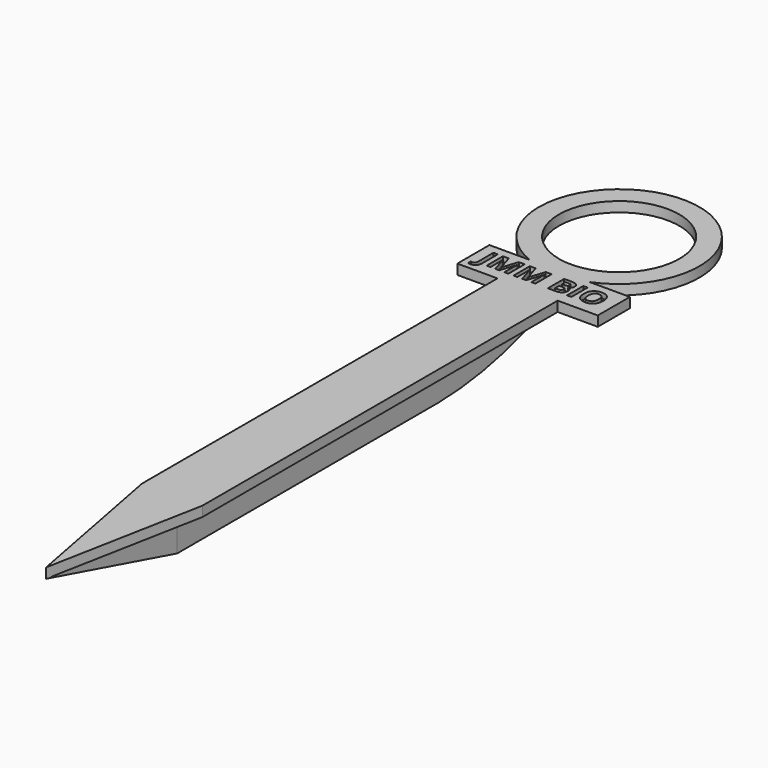
from build123d import *

# Parameters (mm, degrees)
F0_R         = 19.05
F1_DEPTH     = 3.175
F2_W         = 3.175
F2_H         = 153.3009581755
F3_DEPTH     = 12.7
F5_DEPTH     = 128.016
F6_W         = 12.7
F6_H         = 12.7
F7_DEPTH     = 3.175
F8_ANGLE     = 180
F9_TEXT_SIZE = 9.0372655213
F10_DEPTH    = 1.5875


# Not quite as in the source:
# - Text() gives the source's letters only with a copy of the font that has no kerning and outlines rounded to 1/6400 em; it was checked with that copy


with BuildPart() as f1:
    # F0 (on Top) → F1 (new body)
    with BuildSketch(Plane.XY):
        with BuildLine():
            ThreePointArc((-32.8058722675, 92.5149641021), (-42.3308722675, 90.6613942987), (-51.8558722675, 92.5149641021))
            Line((-51.8558722675, 92.5149641021), (-51.8558722675, -60.7859940734))
            Line((-51.8558722675, -60.7859940734), (-42.3308722675, -110.6850358979))
            Line((-42.3308722675, -110.6850358979), (-32.8058722675, -60.7859940734))
            Line((-32.8058722675, -60.7859940734), (-32.8058722675, 92.5149641021))
        make_face()
        with BuildLine():
            Line((-32.8058722675, 92.5149641021), (-51.8558722675, 92.5149641021))
            ThreePointArc((-51.8558722675, 92.5149641021), (-42.3308722675, 90.6613942987), (-32.8058722675, 92.5149641021))
        make_face()
        with BuildLine():
            ThreePointArc((-16.9308722675, 116.0613942987), (-56.5299039246, 137.1219617174), (-51.8558722675, 92.5149641021))
            Line((-51.8558722675, 92.5149641021), (-32.8058722675, 92.5149641021))
            ThreePointArc((-32.8058722675, 92.5149641021), (-21.2703048487, 101.8623626415), (-16.9308722675, 116.0613942987))
        make_face()
        with Locations((-42.3308722675, 116.0613942987)):
            Circle(F0_R, mode=Mode.SUBTRACT)
    extrude(amount=F1_DEPTH)

    # F2 (on face) → F3 (join)
    with BuildSketch(Plane.XY.offset(3.175)):
        with Locations((-42.3308722675, 15.8644850144)):
            Rectangle(F2_W, F2_H)
        Polygon((-40.7433722675, -60.7859940734), (-43.9183722675, -60.7859940734), (-42.3308722675, -110.6850358979), align=None)
    extrude(amount=F3_DEPTH)

    # F4 (on Right) → F5 (cut)
    with BuildSketch(Plane.YZ):
        Polygon((-110.6850358979, 3.175), (-60.7859940734, 15.875), (-110.6850358979, 15.875), align=None)
        with BuildLine():
            ThreePointArc((42.7295640111, 15.875), (68.363979336, 12.4326056643), (92.5149641021, 3.175))
            Line((92.5149641021, 3.175), (92.5149641021, 15.875))
            Line((92.5149641021, 15.875), (42.7295640111, 15.875))
        make_face()
    extrude(amount=-F5_DEPTH, mode=Mode.SUBTRACT)

    # F6 (on face) → F7 (join)
    with BuildSketch(Plane(origin=(0, 0, 0), x_dir=(1, 0, 0), z_dir=(0, 0, -1))):
        with Locations((-26.4558722675, -86.1649641021)):
            Rectangle(F6_W, F6_H)
        with Locations((-58.2058722675, -86.1649641021)):
            Rectangle(F6_W, F6_H)
    extrude(amount=-F7_DEPTH)


with BuildPart() as f1_1:
    # F8: moved
    add(f1.part.rotate(Axis((-20.1058722675, 86.1649641021, 0), (0, -1, 0)), F8_ANGLE))

    # F9 (on face) → F10 (cut)
    with BuildSketch(Plane.XY):
        with Locations((-17.5658722675, 83.4681329268)):
            Text('JMM BIO', F9_TEXT_SIZE, font='Open Sans', font_style=FontStyle.BOLD, text_align=(TextAlign.LEFT, TextAlign.BOTTOM))
    extrude(amount=-F10_DEPTH, mode=Mode.SUBTRACT)


solid = f1_1.part
